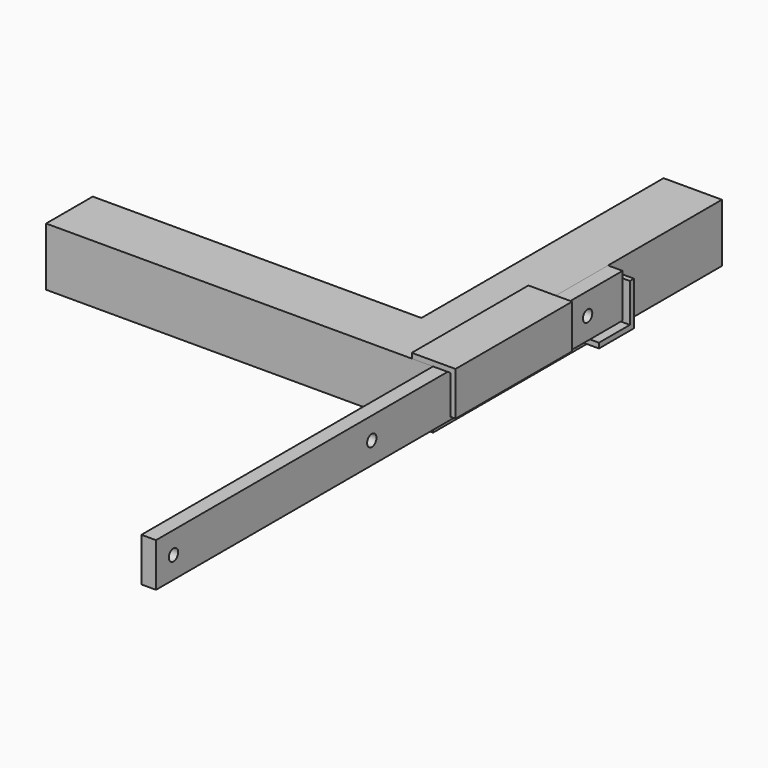
from build123d import *

# Parameters (mm, degrees)
F1_DEPTH = 40
F2_W     = 250
F2_H     = 30
F2_R     = 4
F2_W_2   = 150
F3_DEPTH = 10
F5_DEPTH = 100
F7_DEPTH = 15


with BuildPart() as f1:
    # F0 (on Top) → F1 (new body)
    with BuildSketch(Plane.XY):
        Polygon((974.6156334877, 40), (974.6156334877, 0), (1240, 0), (1240, 247.6407289505), (1200, 247.6407289505), (1200, 40), align=None)
    extrude(amount=F1_DEPTH)


with BuildPart() as f3:
    # F2 (on face) → F3 (new body)
    with BuildSketch(Plane.YZ.offset(1240)):
        with Locations((-125, 25)):
            Rectangle(F2_W, F2_H)
        with Locations((-235, 25)):
            Circle(F2_R, mode=Mode.SUBTRACT)
        with Locations((-65, 25)):
            Circle(F2_R, mode=Mode.SUBTRACT)
        with Locations((75, 25)):
            Rectangle(F2_W_2, F2_H)
        with Locations((70, 25)):
            Circle(F2_R, mode=Mode.SUBTRACT)
        with Locations((120, 25)):
            Circle(F2_R, mode=Mode.SUBTRACT)
    extrude(amount=F3_DEPTH)


with BuildPart() as f5:
    # F4 (on face) → F5 (new body)
    with BuildSketch(Plane.XZ):
        Polygon((1240, 40), (1252, 40), (1251.9164218903, 13.5), (1255.4164218903, 13.5), (1255.4164218903, 43.5), (1225.4164218903, 43.5), (1225.4164218903, 40), align=None)
    extrude(amount=-F5_DEPTH)


with BuildPart() as f7:
    # F6 (on face) → F7 (new body)
    with BuildSketch(Plane.YZ.offset(1240)):
        Polygon((150, 35.5), (150, 10), (150, 9), (123.5, 9), (123.5, 5.5), (153.5, 5.5), (153.5, 35.5), align=None)
    extrude(amount=F7_DEPTH)


solid = Compound([f1.part, f3.part, f5.part, f7.part])
